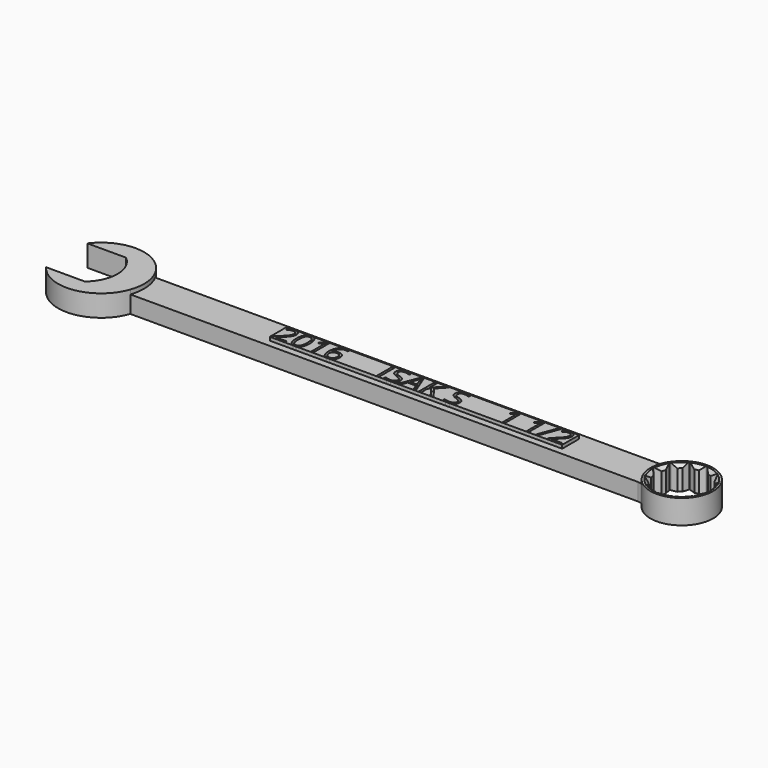
from build123d import *

# Parameters (mm, degrees)
F0_W         = 0.4390429688
F0_H         = 3.7777539063
F0_TEXT_SIZE = 5.2916666667
F1_DEPTH     = 12.7
F2_DEPTH     = 15.875
F0_R         = 19.05
F3_DEPTH     = 17.78
F4_SIZE      = 2.54
F5_R         = 23.1775
F6_DEPTH     = 17.78
F7_DEPTH     = 17.78
F8_COUNT     = 12
F11_DEPTH    = 2.54


# Not quite as in the source:
# - Text() gives the source's letters only with a copy of the font that has no kerning and outlines rounded to 1/6400 em; it was checked with that copy


with BuildPart() as f1:
    # F0 (on Top) → F1 (new body)
    with BuildSketch(Plane.XY):
        with BuildLine():
            ThreePointArc((28.0246586732, -7.9809556568), (31.6571563563, -20.4771515881), (29.9713945913, -33.3809556568))
            Line((29.9713945913, -33.3809556568), (404.6339280202, -33.3809556568))
            ThreePointArc((404.6339280202, -33.3809556568), (406.3354190659, -33.6131596303), (407.9124713773, -34.2927892879))
            Line((407.9124713773, -34.2927892879), (410.7505330951, -36.0037903424))
            ThreePointArc((410.7505330951, -36.0037903424), (406.5998341239, -20.5575243331), (413.8953174208, -6.3240651947))
            Line((413.8953174208, -6.3240651947), (410.0995642824, -7.6337042455))
            ThreePointArc((410.0995642824, -7.6337042455), (409.078462267, -7.8935411268), (408.0284512048, -7.9809556568))
            Line((408.0284512048, -7.9809556568), (28.0246586732, -7.9809556568))
        make_face()
        with BuildLine():
            ThreePointArc((254.0400713214, -25.8320806663), (253.1382651208, -28.1269866729), (250.8660139713, -29.0844430512))
            Line((250.8660139713, -29.0844430512), (144.2758794034, -29.0844430512))
            ThreePointArc((144.2758794034, -29.0844430512), (142.0308153732, -28.1545070815), (141.1008794034, -25.9094430512))
            Line((141.1008794034, -25.9094430512), (141.1008794034, -22.0994430512))
            ThreePointArc((141.1008794034, -22.0994430512), (142.0308153732, -19.854379021), (144.2758794034, -18.9244430512))
            Line((144.2758794034, -18.9244430512), (250.7731515389, -18.9244430512))
            ThreePointArc((250.7731515389, -18.9244430512), (252.9906951605, -19.8271919018), (253.9472088889, -22.0220806663))
            Line((253.9472088889, -22.0220806663), (254.0400713214, -25.8320806663))
        make_face(mode=Mode.SUBTRACT)
        with BuildLine():
            Line((144.2758794034, -29.0844430512), (250.8660139713, -29.0844430512))
            ThreePointArc((250.8660139713, -29.0844430512), (253.1382651208, -28.1269866729), (254.0400713214, -25.8320806663))
            Line((254.0400713214, -25.8320806663), (253.9472088889, -22.0220806663))
            ThreePointArc((253.9472088889, -22.0220806663), (252.9906951605, -19.8271919018), (250.7731515389, -18.9244430512))
            Line((250.7731515389, -18.9244430512), (144.2758794034, -18.9244430512))
            ThreePointArc((144.2758794034, -18.9244430512), (142.0308153732, -19.854379021), (141.1008794034, -22.0994430512))
            Line((141.1008794034, -22.0994430512), (141.1008794034, -25.9094430512))
            ThreePointArc((141.1008794034, -25.9094430512), (142.0308153732, -28.1545070815), (144.2758794034, -29.0844430512))
        make_face()
        with BuildLine():
            Line((147.0176241951, -25.5117412283), (147.0176241951, -25.9094430512))
            Line((147.0176241951, -25.9094430512), (144.5346749764, -25.9094430512))
            Line((144.5346749764, -25.9094430512), (144.5346749764, -25.5398532075))
            Line((144.5346749764, -25.5398532075), (145.5293429451, -24.5402243012))
            add(Edge.make_bspline(
                [(145.5293429451, -24.5402243012), (145.9840955493, -24.0796839366), (146.1287895597, -23.8833134939)],
                knots=[0, 0, 0, 1, 1, 1], degree=2))
            add(Edge.make_bspline(
                [(146.1287895597, -23.8833134939), (146.2734835701, -23.6869430512), (146.3458305753, -23.500907895)],
                knots=[0, 0, 0, 1, 1, 1], degree=2))
            add(Edge.make_bspline(
                [(146.3458305753, -23.500907895), (146.4181775805, -23.3148727387), (146.4181775805, -23.1007256033)],
                knots=[0, 0, 0, 1, 1, 1], degree=2))
            add(Edge.make_bspline(
                [(146.4181775805, -23.1007256033), (146.4181775805, -22.7981084158), (146.234622893, -22.6211683116)],
                knots=[0, 0, 0, 1, 1, 1], degree=2))
            add(Edge.make_bspline(
                [(146.234622893, -22.6211683116), (146.0510682055, -22.4442282075), (145.7252999764, -22.4442282075)],
                knots=[0, 0, 0, 1, 1, 1], degree=2))
            add(Edge.make_bspline(
                [(145.7252999764, -22.4442282075), (145.490482268, -22.4442282075), (145.2796424243, -22.5219495616)],
                knots=[0, 0, 0, 1, 1, 1], degree=2))
            add(Edge.make_bspline(
                [(145.2796424243, -22.5219495616), (145.0688025805, -22.5996709158), (144.8108338305, -22.8038961762)],
                knots=[0, 0, 0, 1, 1, 1], degree=2))
            Line((144.8108338305, -22.8038961762), (144.5834575284, -22.5120276866))
            add(Edge.make_bspline(
                [(144.5834575284, -22.5120276866), (145.1051827889, -22.0779456554), (145.7203390389, -22.0779456554)],
                knots=[0, 0, 0, 1, 1, 1], degree=2))
            add(Edge.make_bspline(
                [(145.7203390389, -22.0779456554), (146.2528129972, -22.0779456554), (146.5550167732, -22.3503838064)],
                knots=[0, 0, 0, 1, 1, 1], degree=2))
            add(Edge.make_bspline(
                [(146.5550167732, -22.3503838064), (146.8572205493, -22.6228219575), (146.8572205493, -23.0825354991)],
                knots=[0, 0, 0, 1, 1, 1], degree=2))
            add(Edge.make_bspline(
                [(146.8572205493, -23.0825354991), (146.8572205493, -23.4422034679), (146.6554757576, -23.7936032075)],
                knots=[0, 0, 0, 1, 1, 1], degree=2))
            add(Edge.make_bspline(
                [(146.6554757576, -23.7936032075), (146.4537309659, -24.1450029471), (145.9014132576, -24.6824378429)],
                knots=[0, 0, 0, 1, 1, 1], degree=2))
            Line((145.9014132576, -24.6824378429), (145.0745903409, -25.4910706554))
            Line((145.0745903409, -25.4910706554), (145.0745903409, -25.5117412283))
            Line((145.0745903409, -25.5117412283), (147.0176241951, -25.5117412283))
        make_face(mode=Mode.SUBTRACT)
        with BuildLine():
            add(Edge.make_bspline(
                [(149.7444861743, -22.5711455252), (150.0636398201, -23.0701331554), (150.0636398201, -24.0151917491)],
                knots=[0, 0, 0, 1, 1, 1], degree=2))
            add(Edge.make_bspline(
                [(150.0636398201, -24.0151917491), (150.0636398201, -24.9949769054), (149.7548214607, -25.4782549002)],
                knots=[0, 0, 0, 1, 1, 1], degree=2))
            add(Edge.make_bspline(
                [(149.7548214607, -25.4782549002), (149.4460031014, -25.961532895), (148.8101762784, -25.961532895)],
                knots=[0, 0, 0, 1, 1, 1], degree=2))
            add(Edge.make_bspline(
                [(148.8101762784, -25.961532895), (148.2008077889, -25.961532895), (147.8828943774, -25.4666793793)],
                knots=[0, 0, 0, 1, 1, 1], degree=2))
            add(Edge.make_bspline(
                [(147.8828943774, -25.4666793793), (147.5649809659, -24.9718258637), (147.5649809659, -24.0151917491)],
                knots=[0, 0, 0, 1, 1, 1], degree=2))
            add(Edge.make_bspline(
                [(147.5649809659, -24.0151917491), (147.5649809659, -23.0287920096), (147.8725590909, -22.5504749523)],
                knots=[0, 0, 0, 1, 1, 1], degree=2))
            add(Edge.make_bspline(
                [(147.8725590909, -22.5504749523), (148.1801372159, -22.072157895), (148.8101762784, -22.072157895)],
                knots=[0, 0, 0, 1, 1, 1], degree=2))
            add(Edge.make_bspline(
                [(148.8101762784, -22.072157895), (149.4253325284, -22.072157895), (149.7444861743, -22.5711455252)],
                knots=[0, 0, 0, 1, 1, 1], degree=2))
        make_face(mode=Mode.SUBTRACT)
        with BuildLine():
            Line((152.1736919034, -22.131689145), (152.1736919034, -25.9094430512))
            Line((152.1736919034, -25.9094430512), (151.7553195076, -25.9094430512))
            Line((151.7553195076, -25.9094430512), (151.7553195076, -23.2173076346))
            add(Edge.make_bspline(
                [(151.7553195076, -23.2173076346), (151.7553195076, -22.8807907075), (151.7759900805, -22.5814808116)],
                knots=[0, 0, 0, 1, 1, 1], degree=2))
            add(Edge.make_bspline(
                [(151.7759900805, -22.5814808116), (151.7222465909, -22.6360511241), (151.6548605232, -22.6951689627)],
                knots=[0, 0, 0, 1, 1, 1], degree=2))
            add(Edge.make_bspline(
                [(151.6548605232, -22.6951689627), (151.5874744555, -22.7542868012), (151.0401176847, -23.1991175304)],
                knots=[0, 0, 0, 1, 1, 1], degree=2))
            Line((151.0401176847, -23.1991175304), (150.8127413826, -22.9047685721))
            Line((150.8127413826, -22.9047685721), (151.8123702889, -22.131689145))
            Line((151.8123702889, -22.131689145), (152.1736919034, -22.131689145))
        make_face(mode=Mode.SUBTRACT)
        with BuildLine():
            add(Edge.make_bspline(
                [(153.9980766691, -25.5208362804), (153.6545317472, -25.0801396658), (153.6545317472, -24.294657895)],
                knots=[0, 0, 0, 1, 1, 1], degree=2))
            add(Edge.make_bspline(
                [(153.6545317472, -24.294657895), (153.6545317472, -23.1809274262), (154.0873735441, -22.6294365408)],
                knots=[0, 0, 0, 1, 1, 1], degree=2))
            add(Edge.make_bspline(
                [(154.0873735441, -22.6294365408), (154.5202153409, -22.0779456554), (155.3677088305, -22.0779456554)],
                knots=[0, 0, 0, 1, 1, 1], degree=2))
            add(Edge.make_bspline(
                [(155.3677088305, -22.0779456554), (155.6595773201, -22.0779456554), (155.8274223722, -22.1267282075)],
                knots=[0, 0, 0, 1, 1, 1], degree=2))
            Line((155.8274223722, -22.1267282075), (155.8274223722, -22.4963180512))
            add(Edge.make_bspline(
                [(155.8274223722, -22.4963180512), (155.6281580493, -22.4318258637), (155.372669768, -22.4318258637)],
                knots=[0, 0, 0, 1, 1, 1], degree=2))
            add(Edge.make_bspline(
                [(155.372669768, -22.4318258637), (154.7649549243, -22.4318258637), (154.4445610441, -22.8100973481)],
                knots=[0, 0, 0, 1, 1, 1], degree=2))
            add(Edge.make_bspline(
                [(154.4445610441, -22.8100973481), (154.1241671639, -23.1883688325), (154.0935747159, -24.0003089366)],
                knots=[0, 0, 0, 1, 1, 1], degree=2))
            Line((154.0935747159, -24.0003089366), (154.1241671639, -24.0003089366))
            add(Edge.make_bspline(
                [(154.1241671639, -24.0003089366), (154.4085942472, -23.5554782075), (155.0237504972, -23.5554782075)],
                knots=[0, 0, 0, 1, 1, 1], degree=2))
            add(Edge.make_bspline(
                [(155.0237504972, -23.5554782075), (155.5330734139, -23.5554782075), (155.8261821378, -23.8630563325)],
                knots=[0, 0, 0, 1, 1, 1], degree=2))
            add(Edge.make_bspline(
                [(155.8261821378, -23.8630563325), (156.1192908618, -24.1706344575), (156.1192908618, -24.6973206554)],
                knots=[0, 0, 0, 1, 1, 1], degree=2))
            add(Edge.make_bspline(
                [(156.1192908618, -24.6973206554), (156.1192908618, -25.286845395), (155.7976567472, -25.624189145)],
                knots=[0, 0, 0, 1, 1, 1], degree=2))
            add(Edge.make_bspline(
                [(155.7976567472, -25.624189145), (155.4760226326, -25.961532895), (154.9278390389, -25.961532895)],
                knots=[0, 0, 0, 1, 1, 1], degree=2))
            add(Edge.make_bspline(
                [(154.9278390389, -25.961532895), (154.3416215909, -25.961532895), (153.9980766691, -25.5208362804)],
                knots=[0, 0, 0, 1, 1, 1], degree=2))
        make_face(mode=Mode.SUBTRACT)
        with Locations((191.4911886482, -24.0205660981)):
            Rectangle(F0_W, F0_H, mode=Mode.SUBTRACT)
        with BuildLine():
            add(Edge.make_bspline(
                [(194.6550265389, -24.2739873221), (194.8782687264, -24.5170732596), (194.8782687264, -24.9040263846)],
                knots=[0, 0, 0, 1, 1, 1], degree=2))
            add(Edge.make_bspline(
                [(194.8782687264, -24.9040263846), (194.8782687264, -25.4026006033), (194.5165337003, -25.6820667491)],
                knots=[0, 0, 0, 1, 1, 1], degree=2))
            add(Edge.make_bspline(
                [(194.5165337003, -25.6820667491), (194.1547986743, -25.961532895), (193.5346814868, -25.961532895)],
                knots=[0, 0, 0, 1, 1, 1], degree=2))
            add(Edge.make_bspline(
                [(193.5346814868, -25.961532895), (192.8633012784, -25.961532895), (192.5011528409, -25.7879000825)],
                knots=[0, 0, 0, 1, 1, 1], degree=2))
            Line((192.5011528409, -25.7879000825), (192.5011528409, -25.3645667491))
            add(Edge.make_bspline(
                [(192.5011528409, -25.3645667491), (192.7343169034, -25.4621318533), (193.0079952889, -25.5191826346)],
                knots=[0, 0, 0, 1, 1, 1], degree=2))
            add(Edge.make_bspline(
                [(193.0079952889, -25.5191826346), (193.2816736743, -25.5762334158), (193.5503911222, -25.5762334158)],
                knots=[0, 0, 0, 1, 1, 1], degree=2))
            add(Edge.make_bspline(
                [(193.5503911222, -25.5762334158), (193.9894340909, -25.5762334158), (194.2118494555, -25.4096285981)],
                knots=[0, 0, 0, 1, 1, 1], degree=2))
            add(Edge.make_bspline(
                [(194.2118494555, -25.4096285981), (194.4342648201, -25.2430237804), (194.4342648201, -24.9453675304)],
                knots=[0, 0, 0, 1, 1, 1], degree=2))
            add(Edge.make_bspline(
                [(194.4342648201, -24.9453675304), (194.4342648201, -24.7494104991), (194.3553032316, -24.6241468273)],
                knots=[0, 0, 0, 1, 1, 1], degree=2))
            add(Edge.make_bspline(
                [(194.3553032316, -24.6241468273), (194.276341643, -24.4988831554), (194.0915467211, -24.3926364106)],
                knots=[0, 0, 0, 1, 1, 1], degree=2))
            add(Edge.make_bspline(
                [(194.0915467211, -24.3926364106), (193.9067517993, -24.2863896658), (193.5297205493, -24.1524443533)],
                knots=[0, 0, 0, 1, 1, 1], degree=2))
            add(Edge.make_bspline(
                [(193.5297205493, -24.1524443533), (193.0030343514, -23.9639287283), (192.7768982836, -23.7055465668)],
                knots=[0, 0, 0, 1, 1, 1], degree=2))
            add(Edge.make_bspline(
                [(192.7768982836, -23.7055465668), (192.5507622159, -23.4471644054), (192.5507622159, -23.0312724783)],
                knots=[0, 0, 0, 1, 1, 1], degree=2))
            add(Edge.make_bspline(
                [(192.5507622159, -23.0312724783), (192.5507622159, -22.5947099783), (192.8785975024, -22.3363278168)],
                knots=[0, 0, 0, 1, 1, 1], degree=2))
            add(Edge.make_bspline(
                [(192.8785975024, -22.3363278168), (193.2064327889, -22.0779456554), (193.7471749764, -22.0779456554)],
                knots=[0, 0, 0, 1, 1, 1], degree=2))
            add(Edge.make_bspline(
                [(193.7471749764, -22.0779456554), (194.3102413826, -22.0779456554), (194.7831840909, -22.2846513846)],
                knots=[0, 0, 0, 1, 1, 1], degree=2))
            Line((194.7831840909, -22.2846513846), (194.6459314868, -22.6666435721))
            add(Edge.make_bspline(
                [(194.6459314868, -22.6666435721), (194.1779497159, -22.4706865408), (193.7364262784, -22.4706865408)],
                knots=[0, 0, 0, 1, 1, 1], degree=2))
            add(Edge.make_bspline(
                [(193.7364262784, -22.4706865408), (193.3875070076, -22.4706865408), (193.1911365649, -22.6203414887)],
                knots=[0, 0, 0, 1, 1, 1], degree=2))
            add(Edge.make_bspline(
                [(193.1911365649, -22.6203414887), (192.9947661222, -22.7699964366), (192.9947661222, -23.0362334158)],
                knots=[0, 0, 0, 1, 1, 1], degree=2))
            add(Edge.make_bspline(
                [(192.9947661222, -23.0362334158), (192.9947661222, -23.2321904471), (193.0671131274, -23.3578675304)],
                knots=[0, 0, 0, 1, 1, 1], degree=2))
            add(Edge.make_bspline(
                [(193.0671131274, -23.3578675304), (193.1394601326, -23.4835446137), (193.3114392993, -23.5881377127)],
                knots=[0, 0, 0, 1, 1, 1], degree=2))
            add(Edge.make_bspline(
                [(193.3114392993, -23.5881377127), (193.4834184659, -23.6927308116), (193.8372986743, -23.8192347179)],
                knots=[0, 0, 0, 1, 1, 1], degree=2))
            add(Edge.make_bspline(
                [(193.8372986743, -23.8192347179), (194.4317843514, -24.0309013846), (194.6550265389, -24.2739873221)],
                knots=[0, 0, 0, 1, 1, 1], degree=2))
        make_face(mode=Mode.SUBTRACT)
        Polygon((198.4807361743, -25.9094430512), (198.0259835701, -25.9094430512), (197.5555213305, -24.7080693533), (196.0416085701, -24.7080693533), (195.5769340909, -25.9094430512), (195.1321033618, -25.9094430512), (196.6253455493, -22.1159795096), (196.994935393, -22.1159795096), align=None, mode=Mode.SUBTRACT)
        Polygon((200.1525721118, -23.7729326346), (201.7284965909, -25.9094430512), (201.211732268, -25.9094430512), (199.8350721118, -24.0772034679), (199.4390239347, -24.4286032075), (199.4390239347, -25.9094430512), (198.9999809659, -25.9094430512), (198.9999809659, -22.131689145), (199.4390239347, -22.131689145), (199.4390239347, -24.0052698741), (201.152201018, -22.131689145), (201.6714458097, -22.131689145), align=None, mode=Mode.SUBTRACT)
        with BuildLine():
            add(Edge.make_bspline(
                [(205.5310551847, -24.2739873221), (205.7542973722, -24.5170732596), (205.7542973722, -24.9040263846)],
                knots=[0, 0, 0, 1, 1, 1], degree=2))
            add(Edge.make_bspline(
                [(205.7542973722, -24.9040263846), (205.7542973722, -25.4026006033), (205.3925623461, -25.6820667491)],
                knots=[0, 0, 0, 1, 1, 1], degree=2))
            add(Edge.make_bspline(
                [(205.3925623461, -25.6820667491), (205.0308273201, -25.961532895), (204.4107101326, -25.961532895)],
                knots=[0, 0, 0, 1, 1, 1], degree=2))
            add(Edge.make_bspline(
                [(204.4107101326, -25.961532895), (203.7393299243, -25.961532895), (203.3771814868, -25.7879000825)],
                knots=[0, 0, 0, 1, 1, 1], degree=2))
            Line((203.3771814868, -25.7879000825), (203.3771814868, -25.3645667491))
            add(Edge.make_bspline(
                [(203.3771814868, -25.3645667491), (203.6103455493, -25.4621318533), (203.8840239347, -25.5191826346)],
                knots=[0, 0, 0, 1, 1, 1], degree=2))
            add(Edge.make_bspline(
                [(203.8840239347, -25.5191826346), (204.1577023201, -25.5762334158), (204.426419768, -25.5762334158)],
                knots=[0, 0, 0, 1, 1, 1], degree=2))
            add(Edge.make_bspline(
                [(204.426419768, -25.5762334158), (204.8654627368, -25.5762334158), (205.0878781014, -25.4096285981)],
                knots=[0, 0, 0, 1, 1, 1], degree=2))
            add(Edge.make_bspline(
                [(205.0878781014, -25.4096285981), (205.3102934659, -25.2430237804), (205.3102934659, -24.9453675304)],
                knots=[0, 0, 0, 1, 1, 1], degree=2))
            add(Edge.make_bspline(
                [(205.3102934659, -24.9453675304), (205.3102934659, -24.7494104991), (205.2313318774, -24.6241468273)],
                knots=[0, 0, 0, 1, 1, 1], degree=2))
            add(Edge.make_bspline(
                [(205.2313318774, -24.6241468273), (205.1523702889, -24.4988831554), (204.967575367, -24.3926364106)],
                knots=[0, 0, 0, 1, 1, 1], degree=2))
            add(Edge.make_bspline(
                [(204.967575367, -24.3926364106), (204.7827804451, -24.2863896658), (204.4057491951, -24.1524443533)],
                knots=[0, 0, 0, 1, 1, 1], degree=2))
            add(Edge.make_bspline(
                [(204.4057491951, -24.1524443533), (203.8790629972, -23.9639287283), (203.6529269295, -23.7055465668)],
                knots=[0, 0, 0, 1, 1, 1], degree=2))
            add(Edge.make_bspline(
                [(203.6529269295, -23.7055465668), (203.4267908618, -23.4471644054), (203.4267908618, -23.0312724783)],
                knots=[0, 0, 0, 1, 1, 1], degree=2))
            add(Edge.make_bspline(
                [(203.4267908618, -23.0312724783), (203.4267908618, -22.5947099783), (203.7546261482, -22.3363278168)],
                knots=[0, 0, 0, 1, 1, 1], degree=2))
            add(Edge.make_bspline(
                [(203.7546261482, -22.3363278168), (204.0824614347, -22.0779456554), (204.6232036222, -22.0779456554)],
                knots=[0, 0, 0, 1, 1, 1], degree=2))
            add(Edge.make_bspline(
                [(204.6232036222, -22.0779456554), (205.1862700284, -22.0779456554), (205.6592127368, -22.2846513846)],
                knots=[0, 0, 0, 1, 1, 1], degree=2))
            Line((205.6592127368, -22.2846513846), (205.5219601326, -22.6666435721))
            add(Edge.make_bspline(
                [(205.5219601326, -22.6666435721), (205.0539783618, -22.4706865408), (204.6124549243, -22.4706865408)],
                knots=[0, 0, 0, 1, 1, 1], degree=2))
            add(Edge.make_bspline(
                [(204.6124549243, -22.4706865408), (204.2635356534, -22.4706865408), (204.0671652107, -22.6203414887)],
                knots=[0, 0, 0, 1, 1, 1], degree=2))
            add(Edge.make_bspline(
                [(204.0671652107, -22.6203414887), (203.870794768, -22.7699964366), (203.870794768, -23.0362334158)],
                knots=[0, 0, 0, 1, 1, 1], degree=2))
            add(Edge.make_bspline(
                [(203.870794768, -23.0362334158), (203.870794768, -23.2321904471), (203.9431417732, -23.3578675304)],
                knots=[0, 0, 0, 1, 1, 1], degree=2))
            add(Edge.make_bspline(
                [(203.9431417732, -23.3578675304), (204.0154887784, -23.4835446137), (204.1874679451, -23.5881377127)],
                knots=[0, 0, 0, 1, 1, 1], degree=2))
            add(Edge.make_bspline(
                [(204.1874679451, -23.5881377127), (204.3594471118, -23.6927308116), (204.7133273201, -23.8192347179)],
                knots=[0, 0, 0, 1, 1, 1], degree=2))
            add(Edge.make_bspline(
                [(204.7133273201, -23.8192347179), (205.3078129972, -24.0309013846), (205.5310551847, -24.2739873221)],
                knots=[0, 0, 0, 1, 1, 1], degree=2))
        make_face(mode=Mode.SUBTRACT)
        with BuildLine():
            Line((238.1053976326, -22.131689145), (238.1053976326, -25.9094430512))
            Line((238.1053976326, -25.9094430512), (237.6870252368, -25.9094430512))
            Line((237.6870252368, -25.9094430512), (237.6870252368, -23.2173076346))
            add(Edge.make_bspline(
                [(237.6870252368, -23.2173076346), (237.6870252368, -22.8807907075), (237.7076958097, -22.5814808116)],
                knots=[0, 0, 0, 1, 1, 1], degree=2))
            add(Edge.make_bspline(
                [(237.7076958097, -22.5814808116), (237.6539523201, -22.6360511241), (237.5865662524, -22.6951689627)],
                knots=[0, 0, 0, 1, 1, 1], degree=2))
            add(Edge.make_bspline(
                [(237.5865662524, -22.6951689627), (237.5191801847, -22.7542868012), (236.9718234139, -23.1991175304)],
                knots=[0, 0, 0, 1, 1, 1], degree=2))
            Line((236.9718234139, -23.1991175304), (236.7444471118, -22.9047685721))
            Line((236.7444471118, -22.9047685721), (237.744076018, -22.131689145))
            Line((237.744076018, -22.131689145), (238.1053976326, -22.131689145))
        make_face(mode=Mode.SUBTRACT)
        with BuildLine():
            Line((242.5057491951, -22.131689145), (242.5057491951, -25.9094430512))
            Line((242.5057491951, -25.9094430512), (242.0873767993, -25.9094430512))
            Line((242.0873767993, -25.9094430512), (242.0873767993, -23.2173076346))
            add(Edge.make_bspline(
                [(242.0873767993, -23.2173076346), (242.0873767993, -22.8807907075), (242.1080473722, -22.5814808116)],
                knots=[0, 0, 0, 1, 1, 1], degree=2))
            add(Edge.make_bspline(
                [(242.1080473722, -22.5814808116), (242.0543038826, -22.6360511241), (241.9869178149, -22.6951689627)],
                knots=[0, 0, 0, 1, 1, 1], degree=2))
            add(Edge.make_bspline(
                [(241.9869178149, -22.6951689627), (241.9195317472, -22.7542868012), (241.3721749764, -23.1991175304)],
                knots=[0, 0, 0, 1, 1, 1], degree=2))
            Line((241.3721749764, -23.1991175304), (241.1447986743, -22.9047685721))
            Line((241.1447986743, -22.9047685721), (242.1444275805, -22.131689145))
            Line((242.1444275805, -22.131689145), (242.5057491951, -22.131689145))
        make_face(mode=Mode.SUBTRACT)
        Polygon((245.1441411222, -22.131689145), (245.572435393, -22.131689145), (244.1643559659, -25.9094430512), (243.7360616951, -25.9094430512), align=None, mode=Mode.SUBTRACT)
        with BuildLine():
            Line((248.3687504972, -25.5117412283), (248.3687504972, -25.9094430512))
            Line((248.3687504972, -25.9094430512), (245.8858012784, -25.9094430512))
            Line((245.8858012784, -25.9094430512), (245.8858012784, -25.5398532075))
            Line((245.8858012784, -25.5398532075), (246.8804692472, -24.5402243012))
            add(Edge.make_bspline(
                [(246.8804692472, -24.5402243012), (247.3352218514, -24.0796839366), (247.4799158618, -23.8833134939)],
                knots=[0, 0, 0, 1, 1, 1], degree=2))
            add(Edge.make_bspline(
                [(247.4799158618, -23.8833134939), (247.6246098722, -23.6869430512), (247.6969568774, -23.500907895)],
                knots=[0, 0, 0, 1, 1, 1], degree=2))
            add(Edge.make_bspline(
                [(247.6969568774, -23.500907895), (247.7693038826, -23.3148727387), (247.7693038826, -23.1007256033)],
                knots=[0, 0, 0, 1, 1, 1], degree=2))
            add(Edge.make_bspline(
                [(247.7693038826, -23.1007256033), (247.7693038826, -22.7981084158), (247.5857491951, -22.6211683116)],
                knots=[0, 0, 0, 1, 1, 1], degree=2))
            add(Edge.make_bspline(
                [(247.5857491951, -22.6211683116), (247.4021945076, -22.4442282075), (247.0764262784, -22.4442282075)],
                knots=[0, 0, 0, 1, 1, 1], degree=2))
            add(Edge.make_bspline(
                [(247.0764262784, -22.4442282075), (246.8416085701, -22.4442282075), (246.6307687264, -22.5219495616)],
                knots=[0, 0, 0, 1, 1, 1], degree=2))
            add(Edge.make_bspline(
                [(246.6307687264, -22.5219495616), (246.4199288826, -22.5996709158), (246.1619601326, -22.8038961762)],
                knots=[0, 0, 0, 1, 1, 1], degree=2))
            Line((246.1619601326, -22.8038961762), (245.9345838305, -22.5120276866))
            add(Edge.make_bspline(
                [(245.9345838305, -22.5120276866), (246.4563090909, -22.0779456554), (247.0714653409, -22.0779456554)],
                knots=[0, 0, 0, 1, 1, 1], degree=2))
            add(Edge.make_bspline(
                [(247.0714653409, -22.0779456554), (247.6039392993, -22.0779456554), (247.9061430753, -22.3503838064)],
                knots=[0, 0, 0, 1, 1, 1], degree=2))
            add(Edge.make_bspline(
                [(247.9061430753, -22.3503838064), (248.2083468514, -22.6228219575), (248.2083468514, -23.0825354991)],
                knots=[0, 0, 0, 1, 1, 1], degree=2))
            add(Edge.make_bspline(
                [(248.2083468514, -23.0825354991), (248.2083468514, -23.4422034679), (248.0066020597, -23.7936032075)],
                knots=[0, 0, 0, 1, 1, 1], degree=2))
            add(Edge.make_bspline(
                [(248.0066020597, -23.7936032075), (247.804857268, -24.1450029471), (247.2525395597, -24.6824378429)],
                knots=[0, 0, 0, 1, 1, 1], degree=2))
            Line((247.2525395597, -24.6824378429), (246.425716643, -25.4910706554))
            Line((246.425716643, -25.4910706554), (246.425716643, -25.5117412283))
            Line((246.425716643, -25.5117412283), (248.3687504972, -25.5117412283))
        make_face(mode=Mode.SUBTRACT)
        Polygon((248.9963090909, -22.131689145), (249.4766932055, -22.131689145), (249.3733403409, -23.4959469575), (249.1021424243, -23.4959469575), align=None, mode=Mode.SUBTRACT)
        Polygon((249.9496359139, -22.131689145), (250.4300200284, -22.131689145), (250.3241866951, -23.4959469575), (250.0554692472, -23.4959469575), align=None, mode=Mode.SUBTRACT)
        with BuildLine():
            add(Edge.make_bspline(
                [(148.1929529711, -22.8175387543), (147.9990629972, -23.1908493012), (147.9990629972, -24.0151917491)],
                knots=[0, 0, 0, 1, 1, 1], degree=2))
            add(Edge.make_bspline(
                [(147.9990629972, -24.0151917491), (147.9990629972, -24.8395341971), (148.1929529711, -25.2157386241)],
                knots=[0, 0, 0, 1, 1, 1], degree=2))
            add(Edge.make_bspline(
                [(148.1929529711, -25.2157386241), (148.3868429451, -25.5919430512), (148.8101762784, -25.5919430512)],
                knots=[0, 0, 0, 1, 1, 1], degree=2))
            add(Edge.make_bspline(
                [(148.8101762784, -25.5919430512), (149.2392973722, -25.5919430512), (149.4315337003, -25.2107776866)],
                knots=[0, 0, 0, 1, 1, 1], degree=2))
            add(Edge.make_bspline(
                [(149.4315337003, -25.2107776866), (149.6237700284, -24.8296123221), (149.6237700284, -24.0151917491)],
                knots=[0, 0, 0, 1, 1, 1], degree=2))
            add(Edge.make_bspline(
                [(149.6237700284, -24.0151917491), (149.6237700284, -23.2015979991), (149.4315337003, -22.8229131033)],
                knots=[0, 0, 0, 1, 1, 1], degree=2))
            add(Edge.make_bspline(
                [(149.4315337003, -22.8229131033), (149.2392973722, -22.4442282075), (148.8101762784, -22.4442282075)],
                knots=[0, 0, 0, 1, 1, 1], degree=2))
            add(Edge.make_bspline(
                [(148.8101762784, -22.4442282075), (148.3868429451, -22.4442282075), (148.1929529711, -22.8175387543)],
                knots=[0, 0, 0, 1, 1, 1], degree=2))
        make_face()
        with BuildLine():
            add(Edge.make_bspline(
                [(154.4900363045, -25.4625452648), (154.6797921639, -25.5969039887), (154.9228781014, -25.5969039887)],
                knots=[0, 0, 0, 1, 1, 1], degree=2))
            add(Edge.make_bspline(
                [(154.9228781014, -25.5969039887), (155.2899874764, -25.5969039887), (155.4925590909, -25.3653935721)],
                knots=[0, 0, 0, 1, 1, 1], degree=2))
            add(Edge.make_bspline(
                [(155.4925590909, -25.3653935721), (155.6951307055, -25.1338831554), (155.6951307055, -24.6973206554)],
                knots=[0, 0, 0, 1, 1, 1], degree=2))
            add(Edge.make_bspline(
                [(155.6951307055, -24.6973206554), (155.6951307055, -24.3227698741), (155.5066150805, -24.1082093273)],
                knots=[0, 0, 0, 1, 1, 1], degree=2))
            add(Edge.make_bspline(
                [(155.5066150805, -24.1082093273), (155.3180994555, -23.8936487804), (154.9435486743, -23.8936487804)],
                knots=[0, 0, 0, 1, 1, 1], degree=2))
            add(Edge.make_bspline(
                [(154.9435486743, -23.8936487804), (154.7112114347, -23.8936487804), (154.5173214607, -23.9895602387)],
                knots=[0, 0, 0, 1, 1, 1], degree=2))
            add(Edge.make_bspline(
                [(154.5173214607, -23.9895602387), (154.3234314868, -24.0854716971), (154.2085031014, -24.2533167491)],
                knots=[0, 0, 0, 1, 1, 1], degree=2))
            add(Edge.make_bspline(
                [(154.2085031014, -24.2533167491), (154.0935747159, -24.4211618012), (154.0935747159, -24.60223602)],
                knots=[0, 0, 0, 1, 1, 1], degree=2))
            add(Edge.make_bspline(
                [(154.0935747159, -24.60223602), (154.0935747159, -24.8684729991), (154.1969275805, -25.09832977)],
                knots=[0, 0, 0, 1, 1, 1], degree=2))
            add(Edge.make_bspline(
                [(154.1969275805, -25.09832977), (154.3002804451, -25.3281865408), (154.4900363045, -25.4625452648)],
                knots=[0, 0, 0, 1, 1, 1], degree=2))
        make_face()
        with BuildLine():
            Line((196.1970512784, -24.3128479991), (197.4190955493, -24.3128479991))
            Line((197.4190955493, -24.3128479991), (196.9792257576, -23.1420667491))
            add(Edge.make_bspline(
                [(196.9792257576, -23.1420667491), (196.8940629972, -22.9196513846), (196.8039392993, -22.5971904471)],
                knots=[0, 0, 0, 1, 1, 1], degree=2))
            add(Edge.make_bspline(
                [(196.8039392993, -22.5971904471), (196.746888518, -22.8452373221), (196.6410551847, -23.1420667491)],
                knots=[0, 0, 0, 1, 1, 1], degree=2))
            Line((196.6410551847, -23.1420667491), (196.1970512784, -24.3128479991))
        make_face()
        with Locations((144.2758794034, -25.9094430512)):
            Text('2016                         ISAK S                      1 1/2"', F0_TEXT_SIZE, font='Open Sans', text_align=(TextAlign.LEFT, TextAlign.BOTTOM))
    extrude(amount=F1_DEPTH)

    # F0 (on Top) → F2 (join)
    with BuildSketch(Plane.XY):
        with BuildLine():
            Line((3.175, -41.9534556568), (-25.4, -41.9534556568))
            ThreePointArc((-25.4, -41.9534556568), (4.8576075582, -54.2796592004), (29.9713945913, -33.3809556568))
            ThreePointArc((29.9713945913, -33.3809556568), (31.6571563563, -20.4771515881), (28.0246586732, -7.9809556568))
            ThreePointArc((28.0246586732, -7.9809556568), (2.4456639896, 8.7522109394), (-25.4, -3.8534556568))
            Line((-25.4, -3.8534556568), (3.175, -3.8534556568))
            ThreePointArc((3.175, -3.8534556568), (12.0699524055, -22.9034556568), (3.175, -41.9534556568))
        make_face()
    extrude(amount=F2_DEPTH)

    # F0 (on Top) → F3 (join)
    with BuildSketch(Plane.XY):
        with BuildLine():
            ThreePointArc((413.8953174208, -6.3240651947), (406.5998341239, -20.5575243331), (410.7505330951, -36.0037903424))
            ThreePointArc((410.7505330951, -36.0037903424), (435.5931010732, -44.0287078572), (450.9261153558, -22.899317003))
            ThreePointArc((450.9261153558, -22.899317003), (437.7810868837, -2.6137373452), (413.8953174208, -6.3240651947))
        make_face()
        with Locations((428.7011153558, -22.899317003)):
            Circle(F0_R, mode=Mode.SUBTRACT)
    extrude(amount=F3_DEPTH)

    # F4
    f4_edges = [f1.edges().sort_by_distance(p)[0] for p in [
        (409.651115, -22.899317, 17.78),
    ]]
    chamfer(f4_edges, length=F4_SIZE)

    # F5 (on face) → F6 (join)
    with BuildSketch(Plane.XY.offset(17.78)):
        with Locations((428.7011153558, -22.899317003)):
            Circle(F5_R)
        with BuildLine():
            ThreePointArc((406.6808373244, -19.8896691131), (407.6216405464, -15.8561382632), (409.2945158604, -12.0672109739))
            ThreePointArc((409.2945158604, -12.0672109739), (411.6413657407, -8.6544734423), (414.5806861024, -5.7364471177))
            ThreePointArc((414.5806861024, -5.7364471177), (418.0103968689, -3.4144725532), (421.811387125, -1.7691899351))
            ThreePointArc((421.811387125, -1.7691899351), (425.8101116486, -0.8631484938), (429.9072262122, -0.7070678695))
            ThreePointArc((429.9072262122, -0.7070678695), (433.9632929919, -1.3062599817), (437.8402711503, -2.6403324193))
            ThreePointArc((437.8402711503, -2.6403324193), (441.3718211102, -4.6399675982), (444.4808765864, -7.2484460846))
            ThreePointArc((444.4808765864, -7.2484460846), (447.1017278191, -10.4346434824), (449.0885246231, -14.0503527492))
            ThreePointArc((449.0885246231, -14.0503527492), (450.3644154805, -17.9342336498), (450.9073457293, -21.9861042147))
            ThreePointArc((450.9073457293, -21.9861042147), (450.9214224537, -22.4426141741), (450.9261153558, -22.899317003))
            ThreePointArc((450.9261153558, -22.899317003), (450.6176350497, -26.5894104307), (449.70075747, -30.1770677594))
            ThreePointArc((449.70075747, -30.1770677594), (448.0145461281, -33.8966810872), (445.6761937607, -37.2449552999))
            ThreePointArc((445.6761937607, -37.2449552999), (442.7646624402, -40.1088279897), (439.3782601188, -42.3916027774))
            ThreePointArc((439.3782601188, -42.3916027774), (435.6396794195, -44.0134580874), (431.6678132357, -44.9254226209))
            ThreePointArc((431.6678132357, -44.9254226209), (427.5784432253, -45.0959436), (423.5271479334, -44.5136799617))
            ThreePointArc((423.5271479334, -44.5136799617), (419.5902103807, -43.1710222972), (415.9724115332, -41.1182830548))
            ThreePointArc((415.9724115332, -41.1182830548), (412.8170374696, -38.4443063792), (410.2117620358, -35.2319744137))
            ThreePointArc((410.2117620358, -35.2319744137), (408.261002646, -31.6258522496), (407.0058384781, -27.7227583266))
            ThreePointArc((407.0058384781, -27.7227583266), (406.4952207125, -23.8206573812), (406.6808373244, -19.8896691131))
        make_face(mode=Mode.SUBTRACT)
    extrude(amount=-F6_DEPTH)


with BuildPart() as f7:
    # F5 (on face) → F7 (new body, through all)
    with BuildSketch(Plane.XY.offset(17.78)):
        with BuildLine():
            Line((429.2230926978, -1.315627799), (426.1875151916, -4.0158767917))
            ThreePointArc((426.1875151916, -4.0158767917), (429.6990692744, -3.8754743844), (433.1766598152, -4.3825137748))
            Line((433.1766598152, -4.3825137748), (430.5105105856, -1.3852706866))
            ThreePointArc((430.5105105856, -1.3852706866), (429.8673216198, -1.3408369325), (429.2230926978, -1.315627799))
        make_face()
        with BuildLine():
            Line((429.9072262122, -0.7070678695), (429.2230926978, -1.315627799))
            ThreePointArc((429.2230926978, -1.315627799), (429.8673216198, -1.3408369325), (430.5105105856, -1.3852706866))
            Line((430.5105105856, -1.3852706866), (429.9072262122, -0.7070678695))
        make_face()
    extrude(amount=-F7_DEPTH)


with BuildPart() as f8_1:
    # F8: instance of F7
    add(f7.part.rotate(Axis((428.7011153558, -22.899317003, 0), (0, 0, -1)), 1 * 360 / F8_COUNT))


with BuildPart() as f8_2:
    # F8: instance of F7
    add(f7.part.rotate(Axis((428.7011153558, -22.899317003, 0), (0, 0, -1)), 2 * 360 / F8_COUNT))


with BuildPart() as f8_3:
    # F8: instance of F7
    add(f7.part.rotate(Axis((428.7011153558, -22.899317003, 0), (0, 0, -1)), 3 * 360 / F8_COUNT))


with BuildPart() as f8_4:
    # F8: instance of F7
    add(f7.part.rotate(Axis((428.7011153558, -22.899317003, 0), (0, 0, -1)), 4 * 360 / F8_COUNT))


with BuildPart() as f8_5:
    # F8: instance of F7
    add(f7.part.rotate(Axis((428.7011153558, -22.899317003, 0), (0, 0, -1)), 5 * 360 / F8_COUNT))


with BuildPart() as f8_6:
    # F8: instance of F7
    add(f7.part.rotate(Axis((428.7011153558, -22.899317003, 0), (0, 0, -1)), 6 * 360 / F8_COUNT))


with BuildPart() as f8_7:
    # F8: instance of F7
    add(f7.part.rotate(Axis((428.7011153558, -22.899317003, 0), (0, 0, -1)), 7 * 360 / F8_COUNT))


with BuildPart() as f8_8:
    # F8: instance of F7
    add(f7.part.rotate(Axis((428.7011153558, -22.899317003, 0), (0, 0, -1)), 8 * 360 / F8_COUNT))


with BuildPart() as f8_9:
    # F8: instance of F7
    add(f7.part.rotate(Axis((428.7011153558, -22.899317003, 0), (0, 0, -1)), 9 * 360 / F8_COUNT))


with BuildPart() as f8_10:
    # F8: instance of F7
    add(f7.part.rotate(Axis((428.7011153558, -22.899317003, 0), (0, 0, -1)), 10 * 360 / F8_COUNT))


with BuildPart() as f8_11:
    # F8: instance of F7
    add(f7.part.rotate(Axis((428.7011153558, -22.899317003, 0), (0, 0, -1)), 11 * 360 / F8_COUNT))


with BuildPart() as f1_1:
    add(f1.part)

    # F9: cut F7, F8_1, F8_2, F8_3, F8_4, F8_5, F8_6, F8_7, F8_8, F8_9, F8_10, F8_11
    add(f7.part, mode=Mode.SUBTRACT)
    add(f8_1.part, mode=Mode.SUBTRACT)
    add(f8_2.part, mode=Mode.SUBTRACT)
    add(f8_3.part, mode=Mode.SUBTRACT)
    add(f8_4.part, mode=Mode.SUBTRACT)
    add(f8_5.part, mode=Mode.SUBTRACT)
    add(f8_6.part, mode=Mode.SUBTRACT)
    add(f8_7.part, mode=Mode.SUBTRACT)
    add(f8_8.part, mode=Mode.SUBTRACT)
    add(f8_9.part, mode=Mode.SUBTRACT)
    add(f8_10.part, mode=Mode.SUBTRACT)
    add(f8_11.part, mode=Mode.SUBTRACT)

    # F10 (on face) → F11 (join)
    with BuildSketch(Plane.XY.offset(12.7)):
        with BuildLine():
            Line((344.7478053731, -28.1739556568), (344.7478053731, -12.8160896817))
            Line((344.7478053731, -12.8160896817), (339.2679984715, -12.8160896817))
            add(Edge.make_bspline(
                [(339.2679984715, -12.8160896817), (340.6239472568, -13.0379191573), (341.4999233434, -13.8276157935)],
                knots=[0.2809046733, 0.2809046733, 0.2809046733, 1, 1, 1], degree=2))
            add(Edge.make_bspline(
                [(341.4999233434, -13.8276157935), (342.7180874089, -14.9257965311), (342.7180874089, -16.7788723736)],
                knots=[0, 0, 0, 1, 1, 1], degree=2))
            add(Edge.make_bspline(
                [(342.7180874089, -16.7788723736), (342.7180874089, -18.2286709194), (341.9048670751, -19.6451407631)],
                knots=[0, 0, 0, 1, 1, 1], degree=2))
            add(Edge.make_bspline(
                [(341.9048670751, -19.6451407631), (341.0916467414, -21.0616106067), (338.8652894342, -23.2279762499)],
                knots=[0, 0, 0, 1, 1, 1], degree=2))
            Line((338.8652894342, -23.2279762499), (335.532419214, -26.4875233253))
            Line((335.532419214, -26.4875233253), (335.532419214, -26.5708450808))
            Line((335.532419214, -26.5708450808), (343.3646642316, -26.5708450808))
            Line((343.3646642316, -26.5708450808), (343.3646642316, -28.1739556568))
            Line((343.3646642316, -28.1739556568), (344.7478053731, -28.1739556568))
        make_face()
        with BuildLine():
            Line((344.7478053731, -12.6890896817), (128.8478053731, -12.6890896817))
            Line((128.8478053731, -12.6890896817), (128.8478053731, -12.8160896817))
            Line((128.8478053731, -12.8160896817), (133.5853386769, -12.8160896817))
            add(Edge.make_bspline(
                [(133.5853386769, -12.8160896817), (134.1185084741, -12.729435056), (134.6703296479, -12.729435056)],
                knots=[0.7774605439, 0.7774605439, 0.7774605439, 1, 1, 1], degree=2))
            add(Edge.make_bspline(
                [(134.6703296479, -12.729435056), (135.2732545683, -12.729435056), (135.8029372634, -12.8160896817)],
                knots=[0, 0, 0, 0.2809046733, 0.2809046733, 0.2809046733], degree=2))
            Line((135.8029372634, -12.8160896817), (145.986278987, -12.8160896817))
            add(Edge.make_bspline(
                [(145.986278987, -12.8160896817), (146.5186988239, -12.7061049644), (147.1252656611, -12.7061049644)],
                knots=[0.7611609757, 0.7611609757, 0.7611609757, 1, 1, 1], degree=2))
            add(Edge.make_bspline(
                [(147.1252656611, -12.7061049644), (147.7051076631, -12.7061049644), (148.2197060383, -12.8160896817)],
                knots=[0, 0, 0, 0.2338397471, 0.2338397471, 0.2338397471], degree=2))
            Line((148.2197060383, -12.8160896817), (172.2744622205, -12.8160896817))
            add(Edge.make_bspline(
                [(172.2744622205, -12.8160896817), (172.8837841166, -12.729435056), (173.5582593782, -12.729435056)],
                knots=[0.802565176, 0.802565176, 0.802565176, 1, 1, 1], degree=2))
            add(Edge.make_bspline(
                [(173.5582593782, -12.729435056), (174.3392643102, -12.729435056), (174.8999608716, -12.8160896817)],
                knots=[0, 0, 0, 0.6638357975, 0.6638357975, 0.6638357975], degree=2))
            Line((174.8999608716, -12.8160896817), (216.226127589, -12.8160896817))
            add(Edge.make_bspline(
                [(216.226127589, -12.8160896817), (216.7834449571, -12.729435056), (217.4121657368, -12.729435056)],
                knots=[0.711555898, 0.711555898, 0.711555898, 1, 1, 1], degree=2))
            add(Edge.make_bspline(
                [(217.4121657368, -12.729435056), (218.1441170333, -12.729435056), (218.838286913, -12.8160896817)],
                knots=[0, 0, 0, 0.3224903099, 0.3224903099, 0.3224903099], degree=2))
            Line((218.838286913, -12.8160896817), (260.0667024667, -12.8160896817))
            add(Edge.make_bspline(
                [(260.0667024667, -12.8160896817), (260.6240198347, -12.729435056), (261.2527406144, -12.729435056)],
                knots=[0.711555898, 0.711555898, 0.711555898, 1, 1, 1], degree=2))
            add(Edge.make_bspline(
                [(261.2527406144, -12.729435056), (261.984691911, -12.729435056), (262.6788617907, -12.8160896817)],
                knots=[0, 0, 0, 0.3224903099, 0.3224903099, 0.3224903099], degree=2))
            Line((262.6788617907, -12.8160896817), (337.050399885, -12.8160896817))
            add(Edge.make_bspline(
                [(337.050399885, -12.8160896817), (337.5835696822, -12.729435056), (338.135390856, -12.729435056)],
                knots=[0.7774605439, 0.7774605439, 0.7774605439, 1, 1, 1], degree=2))
            add(Edge.make_bspline(
                [(338.135390856, -12.729435056), (338.7383157764, -12.729435056), (339.2679984715, -12.8160896817)],
                knots=[0, 0, 0, 0.2809046733, 0.2809046733, 0.2809046733], degree=2))
            Line((339.2679984715, -12.8160896817), (344.7478053731, -12.8160896817))
            Line((344.7478053731, -12.8160896817), (344.7478053731, -12.6890896817))
        make_face()
        with BuildLine():
            Line((133.5853386769, -12.8160896817), (128.8478053731, -12.8160896817))
            Line((128.8478053731, -12.8160896817), (128.8478053731, -28.1739556568))
            Line((128.8478053731, -28.1739556568), (129.890993752, -28.1739556568))
            Line((129.890993752, -28.1739556568), (129.890993752, -26.6841626683))
            Line((129.890993752, -26.6841626683), (133.900436627, -22.654722572))
            add(Edge.make_bspline(
                [(133.900436627, -22.654722572), (135.7335152482, -20.7983138593), (136.3167675367, -20.006757182)],
                knots=[0, 0, 0, 1, 1, 1], degree=2))
            add(Edge.make_bspline(
                [(136.3167675367, -20.006757182), (136.9000198253, -19.2152005046), (137.1916459695, -18.4653047051)],
                knots=[0, 0, 0, 1, 1, 1], degree=2))
            add(Edge.make_bspline(
                [(137.1916459695, -18.4653047051), (137.4832721138, -17.7154089055), (137.4832721138, -16.8521955185)],
                knots=[0, 0, 0, 1, 1, 1], degree=2))
            add(Edge.make_bspline(
                [(137.4832721138, -16.8521955185), (137.4832721138, -15.6323650178), (136.7433749249, -14.9191307907)],
                knots=[0, 0, 0, 1, 1, 1], degree=2))
            add(Edge.make_bspline(
                [(136.7433749249, -14.9191307907), (136.003477736, -14.2058965635), (134.6903268692, -14.2058965635)],
                knots=[0, 0, 0, 1, 1, 1], degree=2))
            add(Edge.make_bspline(
                [(134.6903268692, -14.2058965635), (133.7437917267, -14.2058965635), (132.8939098205, -14.5191863642)],
                knots=[0, 0, 0, 1, 1, 1], degree=2))
            add(Edge.make_bspline(
                [(132.8939098205, -14.5191863642), (132.0440279143, -14.832476165), (131.0041724056, -15.6556951094)],
                knots=[0, 0, 0, 1, 1, 1], degree=2))
            Line((131.0041724056, -15.6556951094), (130.087633095, -14.4791919216))
            add(Edge.make_bspline(
                [(130.087633095, -14.4791919216), (131.7226645794, -13.1188249972), (133.5853386769, -12.8160896817)],
                knots=[0, 0, 0, 0.7774605439, 0.7774605439, 0.7774605439], degree=2))
        make_face()
        with BuildLine():
            Line((129.890993752, -28.1739556568), (128.8478053731, -28.1739556568))
            Line((128.8478053731, -28.1739556568), (128.8478053731, -28.3009556568))
            Line((128.8478053731, -28.3009556568), (146.1722033543, -28.3009556568))
            add(Edge.make_bspline(
                [(146.1722033543, -28.3009556568), (145.9051022417, -28.2519361316), (145.65505833, -28.1739556568)],
                knots=[0.2039489259, 0.2039489259, 0.2039489259, 0.3244428423, 0.3244428423, 0.3244428423], degree=2))
            Line((145.65505833, -28.1739556568), (139.8996030235, -28.1739556568))
            Line((139.8996030235, -28.1739556568), (129.890993752, -28.1739556568))
        make_face()
        with BuildLine():
            Line((344.7478053731, -28.3009556568), (344.7478053731, -28.1739556568))
            Line((344.7478053731, -28.1739556568), (343.3646642316, -28.1739556568))
            Line((343.3646642316, -28.1739556568), (333.3560549601, -28.1739556568))
            Line((333.3560549601, -28.1739556568), (326.4170191615, -28.1739556568))
            Line((326.4170191615, -28.1739556568), (324.6905923874, -28.1739556568))
            Line((324.6905923874, -28.1739556568), (319.7312814996, -28.1739556568))
            Line((319.7312814996, -28.1739556568), (318.0448491681, -28.1739556568))
            Line((318.0448491681, -28.1739556568), (301.9937461872, -28.1739556568))
            Line((301.9937461872, -28.1739556568), (300.3073138557, -28.1739556568))
            Line((300.3073138557, -28.1739556568), (262.3604117209, -28.1739556568))
            add(Edge.make_bspline(
                [(262.3604117209, -28.1739556568), (262.031717543, -28.2519361316), (261.6762473391, -28.3009556568)],
                knots=[0.5682703015, 0.5682703015, 0.5682703015, 0.7286091822, 0.7286091822, 0.7286091822], degree=2))
            Line((261.6762473391, -28.3009556568), (344.7478053731, -28.3009556568))
        make_face()
        with BuildLine():
            add(Edge.make_bspline(
                [(146.1722033543, -28.3009556568), (145.9051022417, -28.2519361316), (145.65505833, -28.1739556568)],
                knots=[0.2039489259, 0.2039489259, 0.2039489259, 0.3244428423, 0.3244428423, 0.3244428423], degree=2))
            Line((146.1722033543, -28.3009556568), (148.1270026884, -28.3009556568))
            add(Edge.make_bspline(
                [(148.6660680686, -28.1739556568), (148.4063335441, -28.2519361316), (148.1270026884, -28.3009556568)],
                knots=[0.6716946069, 0.6716946069, 0.6716946069, 0.7936230252, 0.7936230252, 0.7936230252], degree=2))
            Line((148.6660680686, -28.1739556568), (145.65505833, -28.1739556568))
        make_face()
        with BuildLine():
            Line((148.1270026884, -28.3009556568), (146.1722033543, -28.3009556568))
            add(Edge.make_bspline(
                [(147.1252656611, -28.3839264806), (146.6243007438, -28.3839264806), (146.1722033543, -28.3009556568)],
                knots=[0, 0, 0, 0.2039489259, 0.2039489259, 0.2039489259], degree=2))
            add(Edge.make_bspline(
                [(148.1270026884, -28.3009556568), (147.6542051421, -28.3839264806), (147.1252656611, -28.3839264806)],
                knots=[0.7936230252, 0.7936230252, 0.7936230252, 1, 1, 1], degree=2))
        make_face()
        with BuildLine():
            add(Edge.make_bspline(
                [(261.6762473391, -28.3009556568), (261.0745757488, -28.3839264806), (260.3961929678, -28.3839264806)],
                knots=[0.7286091822, 0.7286091822, 0.7286091822, 1, 1, 1], degree=2))
            Line((261.6762473391, -28.3009556568), (258.6803790273, -28.3009556568))
            add(Edge.make_bspline(
                [(260.3961929678, -28.3839264806), (259.4644024544, -28.3839264806), (258.6803790273, -28.3009556568)],
                knots=[0, 0, 0, 0.3443054145, 0.3443054145, 0.3443054145], degree=2))
        make_face()
        with BuildLine():
            Line((258.6803790273, -28.3009556568), (261.6762473391, -28.3009556568))
            add(Edge.make_bspline(
                [(262.3604117209, -28.1739556568), (262.031717543, -28.2519361316), (261.6762473391, -28.3009556568)],
                knots=[0.5682703015, 0.5682703015, 0.5682703015, 0.7286091822, 0.7286091822, 0.7286091822], degree=2))
            Line((262.3604117209, -28.1739556568), (257.8055481683, -28.1739556568))
            add(Edge.make_bspline(
                [(258.6803790273, -28.3009556568), (258.2171745617, -28.2519361316), (257.8055481683, -28.1739556568)],
                knots=[0.3443054145, 0.3443054145, 0.3443054145, 0.5477225575, 0.5477225575, 0.5477225575], degree=2))
        make_face()
        with BuildLine():
            add(Edge.make_bspline(
                [(148.6660680686, -28.1739556568), (148.4063335441, -28.2519361316), (148.1270026884, -28.3009556568)],
                knots=[0.6716946069, 0.6716946069, 0.6716946069, 0.7936230252, 0.7936230252, 0.7936230252], degree=2))
            Line((148.1270026884, -28.3009556568), (170.8094874911, -28.3009556568))
            add(Edge.make_bspline(
                [(170.8094874911, -28.3009556568), (170.5347644957, -28.2519361316), (170.2759890402, -28.1739556568)],
                knots=[0.2161174802, 0.2161174802, 0.2161174802, 0.3438006316, 0.3438006316, 0.3438006316], degree=2))
            Line((170.2759890402, -28.1739556568), (160.6833817172, -28.1739556568))
            Line((160.6833817172, -28.1739556568), (158.9969493858, -28.1739556568))
            Line((158.9969493858, -28.1739556568), (148.6660680686, -28.1739556568))
        make_face()
        with BuildLine():
            Line((217.8356724615, -28.3009556568), (258.6803790273, -28.3009556568))
            add(Edge.make_bspline(
                [(258.6803790273, -28.3009556568), (258.2171745617, -28.2519361316), (257.8055481683, -28.1739556568)],
                knots=[0.3443054145, 0.3443054145, 0.3443054145, 0.5477225575, 0.5477225575, 0.5477225575], degree=2))
            Line((257.8055481683, -28.1739556568), (249.5843619732, -28.1739556568))
            Line((249.5843619732, -28.1739556568), (247.5013180855, -28.1739556568))
            Line((247.5013180855, -28.1739556568), (240.3556443332, -28.1739556568))
            Line((240.3556443332, -28.1739556568), (238.5858902462, -28.1739556568))
            Line((238.5858902462, -28.1739556568), (236.4928477479, -28.1739556568))
            Line((236.4928477479, -28.1739556568), (234.6597691267, -28.1739556568))
            Line((234.6597691267, -28.1739556568), (224.7878075342, -28.1739556568))
            Line((224.7878075342, -28.1739556568), (222.9947233557, -28.1739556568))
            Line((222.9947233557, -28.1739556568), (218.5198368433, -28.1739556568))
            add(Edge.make_bspline(
                [(218.5198368433, -28.1739556568), (218.1911426653, -28.2519361316), (217.8356724615, -28.3009556568)],
                knots=[0.5682703015, 0.5682703015, 0.5682703015, 0.7286091822, 0.7286091822, 0.7286091822], degree=2))
        make_face()
        with BuildLine():
            add(Edge.make_bspline(
                [(170.8094874911, -28.3009556568), (170.5347644957, -28.2519361316), (170.2759890402, -28.1739556568)],
                knots=[0.2161174802, 0.2161174802, 0.2161174802, 0.3438006316, 0.3438006316, 0.3438006316], degree=2))
            Line((170.8094874911, -28.3009556568), (172.8211066602, -28.3009556568))
            add(Edge.make_bspline(
                [(173.3807718936, -28.1739556568), (173.1106639095, -28.2519361316), (172.8211066602, -28.3009556568)],
                knots=[0.607047376, 0.607047376, 0.607047376, 0.7529849479, 0.7529849479, 0.7529849479], degree=2))
            Line((173.3807718936, -28.1739556568), (170.2759890402, -28.1739556568))
        make_face()
        with BuildLine():
            Line((172.8211066602, -28.3009556568), (170.8094874911, -28.3009556568))
            add(Edge.make_bspline(
                [(171.785172421, -28.3839264806), (171.2744857377, -28.3839264806), (170.8094874911, -28.3009556568)],
                knots=[0, 0, 0, 0.2161174802, 0.2161174802, 0.2161174802], degree=2))
            add(Edge.make_bspline(
                [(172.8211066602, -28.3009556568), (172.3309998418, -28.3839264806), (171.785172421, -28.3839264806)],
                knots=[0.7529849479, 0.7529849479, 0.7529849479, 1, 1, 1], degree=2))
        make_face()
        with BuildLine():
            add(Edge.make_bspline(
                [(217.8356724615, -28.3009556568), (217.2340008712, -28.3839264806), (216.5556180901, -28.3839264806)],
                knots=[0.7286091822, 0.7286091822, 0.7286091822, 1, 1, 1], degree=2))
            Line((217.8356724615, -28.3009556568), (214.8398041496, -28.3009556568))
            add(Edge.make_bspline(
                [(216.5556180901, -28.3839264806), (215.6238275767, -28.3839264806), (214.8398041496, -28.3009556568)],
                knots=[0, 0, 0, 0.3443054145, 0.3443054145, 0.3443054145], degree=2))
        make_face()
        with BuildLine():
            Line((214.8398041496, -28.3009556568), (217.8356724615, -28.3009556568))
            add(Edge.make_bspline(
                [(218.5198368433, -28.1739556568), (218.1911426653, -28.2519361316), (217.8356724615, -28.3009556568)],
                knots=[0.5682703015, 0.5682703015, 0.5682703015, 0.7286091822, 0.7286091822, 0.7286091822], degree=2))
            Line((218.5198368433, -28.1739556568), (213.9649732906, -28.1739556568))
            add(Edge.make_bspline(
                [(214.8398041496, -28.3009556568), (214.376599684, -28.2519361316), (213.9649732906, -28.1739556568)],
                knots=[0.3443054145, 0.3443054145, 0.3443054145, 0.5477225575, 0.5477225575, 0.5477225575], degree=2))
        make_face()
        with BuildLine():
            add(Edge.make_bspline(
                [(173.3807718936, -28.1739556568), (173.1106639095, -28.2519361316), (172.8211066602, -28.3009556568)],
                knots=[0.607047376, 0.607047376, 0.607047376, 0.7529849479, 0.7529849479, 0.7529849479], degree=2))
            Line((172.8211066602, -28.3009556568), (214.8398041496, -28.3009556568))
            add(Edge.make_bspline(
                [(214.8398041496, -28.3009556568), (214.376599684, -28.2519361316), (213.9649732906, -28.1739556568)],
                knots=[0.3443054145, 0.3443054145, 0.3443054145, 0.5477225575, 0.5477225575, 0.5477225575], degree=2))
            Line((213.9649732906, -28.1739556568), (209.2033063842, -28.1739556568))
            Line((209.2033063842, -28.1739556568), (207.4335522972, -28.1739556568))
            Line((207.4335522972, -28.1739556568), (173.3807718936, -28.1739556568))
        make_face()
        with BuildLine():
            Line((145.986278987, -12.8160896817), (135.8029372634, -12.8160896817))
            add(Edge.make_bspline(
                [(135.8029372634, -12.8160896817), (137.1588860487, -13.0379191573), (138.0348621353, -13.8276157935)],
                knots=[0.2809046733, 0.2809046733, 0.2809046733, 1, 1, 1], degree=2))
            add(Edge.make_bspline(
                [(138.0348621353, -13.8276157935), (139.2530262008, -14.9257965311), (139.2530262008, -16.7788723736)],
                knots=[0, 0, 0, 1, 1, 1], degree=2))
            add(Edge.make_bspline(
                [(139.2530262008, -16.7788723736), (139.2530262008, -18.2286709194), (138.439805867, -19.6451407631)],
                knots=[0, 0, 0, 1, 1, 1], degree=2))
            add(Edge.make_bspline(
                [(138.439805867, -19.6451407631), (137.6265855333, -21.0616106067), (135.4002282261, -23.2279762499)],
                knots=[0, 0, 0, 1, 1, 1], degree=2))
            Line((135.4002282261, -23.2279762499), (132.0673580059, -26.4875233253))
            Line((132.0673580059, -26.4875233253), (132.0673580059, -26.5708450808))
            Line((132.0673580059, -26.5708450808), (139.8996030235, -26.5708450808))
            Line((139.8996030235, -26.5708450808), (139.8996030235, -28.1739556568))
            Line((139.8996030235, -28.1739556568), (145.65505833, -28.1739556568))
            add(Edge.make_bspline(
                [(145.65505833, -28.1739556568), (144.2531705051, -27.7367529372), (143.3874517091, -26.3892036538)],
                knots=[0.3244428423, 0.3244428423, 0.3244428423, 1, 1, 1], degree=2))
            add(Edge.make_bspline(
                [(143.3874517091, -26.3892036538), (142.1059631094, -24.394480827), (142.1059631094, -20.5383499821)],
                knots=[0, 0, 0, 1, 1, 1], degree=2))
            add(Edge.make_bspline(
                [(142.1059631094, -20.5383499821), (142.1059631094, -16.5622358093), (143.3457908313, -14.6341703868)],
                knots=[0, 0, 0, 1, 1, 1], degree=2))
            add(Edge.make_bspline(
                [(143.3457908313, -14.6341703868), (144.2894993099, -13.1666022286), (145.986278987, -12.8160896817)],
                knots=[0, 0, 0, 0.7611609757, 0.7611609757, 0.7611609757], degree=2))
        make_face()
        with BuildLine():
            Line((172.2744622205, -12.8160896817), (148.2197060383, -12.8160896817))
            add(Edge.make_bspline(
                [(148.2197060383, -12.8160896817), (149.9057531114, -13.1764472335), (150.89140901, -14.7174921424)],
                knots=[0.2338397471, 0.2338397471, 0.2338397471, 1, 1, 1], degree=2))
            add(Edge.make_bspline(
                [(150.89140901, -14.7174921424), (152.1778969151, -16.7288793203), (152.1778969151, -20.5383499821)],
                knots=[0, 0, 0, 1, 1, 1], degree=2))
            add(Edge.make_bspline(
                [(152.1778969151, -20.5383499821), (152.1778969151, -24.4878011931), (150.9330698878, -26.4358638369)],
                knots=[0, 0, 0, 1, 1, 1], degree=2))
            add(Edge.make_bspline(
                [(150.9330698878, -26.4358638369), (150.096926287, -27.7443670086), (148.6660680686, -28.1739556568)],
                knots=[0, 0, 0, 0.6716946069, 0.6716946069, 0.6716946069], degree=2))
            Line((148.6660680686, -28.1739556568), (158.9969493858, -28.1739556568))
            Line((158.9969493858, -28.1739556568), (158.9969493858, -17.3221302195))
            add(Edge.make_bspline(
                [(158.9969493858, -17.3221302195), (158.9969493858, -15.9656520399), (159.0802711413, -14.7591530201)],
                knots=[0, 0, 0, 1, 1, 1], degree=2))
            add(Edge.make_bspline(
                [(159.0802711413, -14.7591530201), (158.863634577, -14.9791224546), (158.592005654, -15.2174226754)],
                knots=[0, 0, 0, 1, 1, 1], degree=2))
            add(Edge.make_bspline(
                [(158.592005654, -15.2174226754), (158.3203767311, -15.4557228962), (156.1140166452, -17.2488070747)],
                knots=[0, 0, 0, 1, 1, 1], degree=2))
            Line((156.1140166452, -17.2488070747), (155.1974773346, -16.0623052762))
            Line((155.1974773346, -16.0623052762), (159.226917431, -12.9460716203))
            Line((159.226917431, -12.9460716203), (160.6833817172, -12.9460716203))
            Line((160.6833817172, -12.9460716203), (160.6833817172, -28.1739556568))
            Line((160.6833817172, -28.1739556568), (170.2759890402, -28.1739556568))
            add(Edge.make_bspline(
                [(170.2759890402, -28.1739556568), (168.9460697154, -27.773192222), (168.0373598583, -26.6075066532)],
                knots=[0.3438006316, 0.3438006316, 0.3438006316, 1, 1, 1], degree=2))
            add(Edge.make_bspline(
                [(168.0373598583, -26.6075066532), (166.6525522818, -24.8310868258), (166.6525522818, -21.6648601165)],
                knots=[0, 0, 0, 1, 1, 1], degree=2))
            add(Edge.make_bspline(
                [(166.6525522818, -21.6648601165), (166.6525522818, -17.1754839298), (168.3973098421, -14.9524594929)],
                knots=[0, 0, 0, 1, 1, 1], degree=2))
            add(Edge.make_bspline(
                [(168.3973098421, -14.9524594929), (169.7975915005, -13.1683374945), (172.2744622205, -12.8160896817)],
                knots=[0, 0, 0, 0.802565176, 0.802565176, 0.802565176], degree=2))
        make_face()
        with BuildLine():
            Line((216.226127589, -12.8160896817), (174.8999608716, -12.8160896817))
            add(Edge.make_bspline(
                [(174.8999608716, -12.8160896817), (175.1838957138, -12.859971291), (175.4113352207, -12.926074399)],
                knots=[0.6638357975, 0.6638357975, 0.6638357975, 1, 1, 1], degree=2))
            Line((175.4113352207, -12.926074399), (175.4113352207, -14.4158673874))
            add(Edge.make_bspline(
                [(175.4113352207, -14.4158673874), (174.6081134976, -14.1559035102), (173.5782565995, -14.1559035102)],
                knots=[0, 0, 0, 1, 1, 1], degree=2))
            add(Edge.make_bspline(
                [(173.5782565995, -14.1559035102), (171.1285969876, -14.1559035102), (169.8371097773, -15.680691636)],
                knots=[0, 0, 0, 1, 1, 1], degree=2))
            add(Edge.make_bspline(
                [(169.8371097773, -15.680691636), (168.5456225669, -17.2054797618), (168.4223063687, -20.4783583181)],
                knots=[0, 0, 0, 1, 1, 1], degree=2))
            Line((168.4223063687, -20.4783583181), (168.5456225669, -20.4783583181))
            add(Edge.make_bspline(
                [(168.5456225669, -20.4783583181), (169.6921299227, -18.6852741396), (172.1717853666, -18.6852741396)],
                knots=[0, 0, 0, 1, 1, 1], degree=2))
            add(Edge.make_bspline(
                [(172.1717853666, -18.6852741396), (174.2248334223, -18.6852741396), (175.4063359154, -19.9251018616)],
                knots=[0, 0, 0, 1, 1, 1], degree=2))
            add(Edge.make_bspline(
                [(175.4063359154, -19.9251018616), (176.5878384085, -21.1649295835), (176.5878384085, -23.2879679138)],
                knots=[0, 0, 0, 1, 1, 1], degree=2))
            add(Edge.make_bspline(
                [(176.5878384085, -23.2879679138), (176.5878384085, -25.6643043809), (175.2913518928, -27.0241154308)],
                knots=[0, 0, 0, 1, 1, 1], degree=2))
            add(Edge.make_bspline(
                [(175.2913518928, -27.0241154308), (174.5043231554, -27.8495851605), (173.3807718936, -28.1739556568)],
                knots=[0, 0, 0, 0.607047376, 0.607047376, 0.607047376], degree=2))
            Line((173.3807718936, -28.1739556568), (207.4335522972, -28.1739556568))
            Line((207.4335522972, -28.1739556568), (207.4335522972, -12.9460716203))
            Line((207.4335522972, -12.9460716203), (209.2033063842, -12.9460716203))
            Line((209.2033063842, -12.9460716203), (209.2033063842, -28.1739556568))
            Line((209.2033063842, -28.1739556568), (213.9649732906, -28.1739556568))
            add(Edge.make_bspline(
                [(213.9649732906, -28.1739556568), (213.0497636393, -28.0005739585), (212.3895303148, -27.6840237344)],
                knots=[0.5477225575, 0.5477225575, 0.5477225575, 1, 1, 1], degree=2))
            Line((212.3895303148, -27.6840237344), (212.3895303148, -25.9775941816))
            add(Edge.make_bspline(
                [(212.3895303148, -25.9775941816), (213.3293997169, -26.3708728676), (214.4325797598, -26.6008409128)],
                knots=[0, 0, 0, 1, 1, 1], degree=2))
            add(Edge.make_bspline(
                [(214.4325797598, -26.6008409128), (215.5357598027, -26.830808958), (216.6189426243, -26.830808958)],
                knots=[0, 0, 0, 1, 1, 1], degree=2))
            add(Edge.make_bspline(
                [(216.6189426243, -26.830808958), (218.3886967113, -26.830808958), (219.2852388006, -26.1592356086)],
                knots=[0, 0, 0, 1, 1, 1], degree=2))
            add(Edge.make_bspline(
                [(219.2852388006, -26.1592356086), (220.1817808898, -25.4876622592), (220.1817808898, -24.2878289799)],
                knots=[0, 0, 0, 1, 1, 1], degree=2))
            add(Edge.make_bspline(
                [(220.1817808898, -24.2878289799), (220.1817808898, -23.4979387377), (219.8634917838, -22.9930088993)],
                knots=[0, 0, 0, 1, 1, 1], degree=2))
            add(Edge.make_bspline(
                [(219.8634917838, -22.9930088993), (219.5452026777, -22.488079061), (218.8003061835, -22.0598052376)],
                knots=[0, 0, 0, 1, 1, 1], degree=2))
            add(Edge.make_bspline(
                [(218.8003061835, -22.0598052376), (218.0554096893, -21.6315314143), (216.5356208688, -21.0916064387)],
                knots=[0, 0, 0, 1, 1, 1], degree=2))
            add(Edge.make_bspline(
                [(216.5356208688, -21.0916064387), (214.4125825385, -20.3317120284), (213.5010425332, -19.2901900846)],
                knots=[0, 0, 0, 1, 1, 1], degree=2))
            add(Edge.make_bspline(
                [(213.5010425332, -19.2901900846), (212.589502528, -18.2486681408), (212.589502528, -16.5722344199)],
                knots=[0, 0, 0, 1, 1, 1], degree=2))
            add(Edge.make_bspline(
                [(212.589502528, -16.5722344199), (212.589502528, -14.8124789436), (213.9109855703, -13.7709569998)],
                knots=[0, 0, 0, 1, 1, 1], degree=2))
            add(Edge.make_bspline(
                [(213.9109855703, -13.7709569998), (214.8512946232, -13.0298559178), (216.226127589, -12.8160896817)],
                knots=[0, 0, 0, 0.711555898, 0.711555898, 0.711555898], degree=2))
        make_face()
        with BuildLine():
            add(Edge.make_bspline(
                [(257.751560448, -13.7709569998), (258.6918695008, -13.0298559178), (260.0667024667, -12.8160896817)],
                knots=[0, 0, 0, 0.711555898, 0.711555898, 0.711555898], degree=2))
            Line((260.0667024667, -12.8160896817), (218.838286913, -12.8160896817))
            add(Edge.make_bspline(
                [(218.838286913, -12.8160896817), (220.2966464531, -12.9981396435), (221.5882521228, -13.562652611)],
                knots=[0.3224903099, 0.3224903099, 0.3224903099, 1, 1, 1], degree=2))
            Line((221.5882521228, -13.562652611), (221.0349956662, -15.1024386528))
            add(Edge.make_bspline(
                [(221.0349956662, -15.1024386528), (219.1485911215, -14.3125484106), (217.3688384239, -14.3125484106)],
                knots=[0, 0, 0, 1, 1, 1], degree=2))
            add(Edge.make_bspline(
                [(217.3688384239, -14.3125484106), (215.9623671909, -14.3125484106), (215.1708105136, -14.9157979205)],
                knots=[0, 0, 0, 1, 1, 1], degree=2))
            add(Edge.make_bspline(
                [(215.1708105136, -14.9157979205), (214.3792538363, -15.5190474303), (214.3792538363, -16.5922316413)],
                knots=[0, 0, 0, 1, 1, 1], degree=2))
            add(Edge.make_bspline(
                [(214.3792538363, -16.5922316413), (214.3792538363, -17.3821218835), (214.6708799806, -17.888718157)],
                knots=[0, 0, 0, 1, 1, 1], degree=2))
            add(Edge.make_bspline(
                [(214.6708799806, -17.888718157), (214.9625061248, -18.3953144304), (215.6557431307, -18.8169225133)],
                knots=[0, 0, 0, 1, 1, 1], degree=2))
            add(Edge.make_bspline(
                [(215.6557431307, -18.8169225133), (216.3489801365, -19.2385305962), (217.7754485908, -19.7484597399)],
                knots=[0, 0, 0, 1, 1, 1], degree=2))
            add(Edge.make_bspline(
                [(217.7754485908, -19.7484597399), (220.1717822792, -20.6016745163), (221.0716572386, -21.581538361)],
                knots=[0, 0, 0, 1, 1, 1], degree=2))
            add(Edge.make_bspline(
                [(221.0716572386, -21.581538361), (221.9715321981, -22.5614022058), (221.9715321981, -24.1211854689)],
                knots=[0, 0, 0, 1, 1, 1], degree=2))
            add(Edge.make_bspline(
                [(221.9715321981, -24.1211854689), (221.9715321981, -26.1309062117), (220.5134014767, -27.2574163462)],
                knots=[0, 0, 0, 1, 1, 1], degree=2))
            add(Edge.make_bspline(
                [(220.5134014767, -27.2574163462), (219.684789092, -27.8975786), (218.5198368433, -28.1739556568)],
                knots=[0, 0, 0, 0.5682703015, 0.5682703015, 0.5682703015], degree=2))
            Line((218.5198368433, -28.1739556568), (222.9947233557, -28.1739556568))
            Line((222.9947233557, -28.1739556568), (229.0138869736, -12.8827470861))
            Line((229.0138869736, -12.8827470861), (230.503679962, -12.8827470861))
            Line((230.503679962, -12.8827470861), (236.4928477479, -28.1739556568))
            Line((236.4928477479, -28.1739556568), (238.5858902462, -28.1739556568))
            Line((238.5858902462, -28.1739556568), (238.5858902462, -12.9460716203))
            Line((238.5858902462, -12.9460716203), (240.3556443332, -12.9460716203))
            Line((240.3556443332, -12.9460716203), (240.3556443332, -20.4983555394))
            Line((240.3556443332, -20.4983555394), (247.2613514296, -12.9460716203))
            Line((247.2613514296, -12.9460716203), (249.354393928, -12.9460716203))
            Line((249.354393928, -12.9460716203), (243.2319113333, -19.5618190075))
            Line((243.2319113333, -19.5618190075), (249.5843619732, -28.1739556568))
            Line((249.5843619732, -28.1739556568), (257.8055481683, -28.1739556568))
            add(Edge.make_bspline(
                [(257.8055481683, -28.1739556568), (256.8903385169, -28.0005739585), (256.2301051924, -27.6840237344)],
                knots=[0.5477225575, 0.5477225575, 0.5477225575, 1, 1, 1], degree=2))
            Line((256.2301051924, -27.6840237344), (256.2301051924, -25.9775941816))
            add(Edge.make_bspline(
                [(256.2301051924, -25.9775941816), (257.1699745946, -26.3708728676), (258.2731546375, -26.6008409128)],
                knots=[0, 0, 0, 1, 1, 1], degree=2))
            add(Edge.make_bspline(
                [(258.2731546375, -26.6008409128), (259.3763346804, -26.830808958), (260.459517502, -26.830808958)],
                knots=[0, 0, 0, 1, 1, 1], degree=2))
            add(Edge.make_bspline(
                [(260.459517502, -26.830808958), (262.229271589, -26.830808958), (263.1258136782, -26.1592356086)],
                knots=[0, 0, 0, 1, 1, 1], degree=2))
            add(Edge.make_bspline(
                [(263.1258136782, -26.1592356086), (264.0223557675, -25.4876622592), (264.0223557675, -24.2878289799)],
                knots=[0, 0, 0, 1, 1, 1], degree=2))
            add(Edge.make_bspline(
                [(264.0223557675, -24.2878289799), (264.0223557675, -23.4979387377), (263.7040666614, -22.9930088993)],
                knots=[0, 0, 0, 1, 1, 1], degree=2))
            add(Edge.make_bspline(
                [(263.7040666614, -22.9930088993), (263.3857775554, -22.488079061), (262.6408810612, -22.0598052376)],
                knots=[0, 0, 0, 1, 1, 1], degree=2))
            add(Edge.make_bspline(
                [(262.6408810612, -22.0598052376), (261.8959845669, -21.6315314143), (260.3761957465, -21.0916064387)],
                knots=[0, 0, 0, 1, 1, 1], degree=2))
            add(Edge.make_bspline(
                [(260.3761957465, -21.0916064387), (258.2531574162, -20.3317120284), (257.3416174109, -19.2901900846)],
                knots=[0, 0, 0, 1, 1, 1], degree=2))
            add(Edge.make_bspline(
                [(257.3416174109, -19.2901900846), (256.4300774057, -18.2486681408), (256.4300774057, -16.5722344199)],
                knots=[0, 0, 0, 1, 1, 1], degree=2))
            add(Edge.make_bspline(
                [(256.4300774057, -16.5722344199), (256.4300774057, -14.8124789436), (257.751560448, -13.7709569998)],
                knots=[0, 0, 0, 1, 1, 1], degree=2))
        make_face()
        with BuildLine():
            Line((227.2874601995, -21.7381832614), (232.213442385, -21.7381832614))
            Line((232.213442385, -21.7381832614), (230.4403554279, -17.0188390295))
            add(Edge.make_bspline(
                [(230.4403554279, -17.0188390295), (230.0970697952, -16.1222969402), (229.7337869412, -14.8224775543)],
                knots=[0, 0, 0, 1, 1, 1], degree=2))
            add(Edge.make_bspline(
                [(229.7337869412, -14.8224775543), (229.503818896, -15.8223386204), (229.0772115078, -17.0188390295)],
                knots=[0, 0, 0, 1, 1, 1], degree=2))
            Line((229.0772115078, -17.0188390295), (227.2874601995, -21.7381832614))
        make_face()
        Polygon((226.6608805981, -23.3312952267), (224.7878075342, -28.1739556568), (234.6597691267, -28.1739556568), (232.7633659714, -23.3312952267), align=None)
        Polygon((240.3556443332, -28.1739556568), (247.5013180855, -28.1739556568), (241.9520891687, -20.7883152486), (240.3556443332, -22.2047850922), align=None)
        with BuildLine():
            add(Edge.make_bspline(
                [(333.5526943031, -14.4791919216), (335.1877257875, -13.1188249972), (337.050399885, -12.8160896817)],
                knots=[0, 0, 0, 0.7774605439, 0.7774605439, 0.7774605439], degree=2))
            Line((337.050399885, -12.8160896817), (262.6788617907, -12.8160896817))
            add(Edge.make_bspline(
                [(262.6788617907, -12.8160896817), (264.1372213308, -12.9981396435), (265.4288270004, -13.562652611)],
                knots=[0.3224903099, 0.3224903099, 0.3224903099, 1, 1, 1], degree=2))
            Line((265.4288270004, -13.562652611), (264.8755705439, -15.1024386528))
            add(Edge.make_bspline(
                [(264.8755705439, -15.1024386528), (262.9891659992, -14.3125484106), (261.2094133016, -14.3125484106)],
                knots=[0, 0, 0, 1, 1, 1], degree=2))
            add(Edge.make_bspline(
                [(261.2094133016, -14.3125484106), (259.8029420686, -14.3125484106), (259.0113853913, -14.9157979205)],
                knots=[0, 0, 0, 1, 1, 1], degree=2))
            add(Edge.make_bspline(
                [(259.0113853913, -14.9157979205), (258.219828714, -15.5190474303), (258.219828714, -16.5922316413)],
                knots=[0, 0, 0, 1, 1, 1], degree=2))
            add(Edge.make_bspline(
                [(258.219828714, -16.5922316413), (258.219828714, -17.3821218835), (258.5114548582, -17.888718157)],
                knots=[0, 0, 0, 1, 1, 1], degree=2))
            add(Edge.make_bspline(
                [(258.5114548582, -17.888718157), (258.8030810025, -18.3953144304), (259.4963180083, -18.8169225133)],
                knots=[0, 0, 0, 1, 1, 1], degree=2))
            add(Edge.make_bspline(
                [(259.4963180083, -18.8169225133), (260.1895550141, -19.2385305962), (261.6160234684, -19.7484597399)],
                knots=[0, 0, 0, 1, 1, 1], degree=2))
            add(Edge.make_bspline(
                [(261.6160234684, -19.7484597399), (264.0123571568, -20.6016745163), (264.9122321163, -21.581538361)],
                knots=[0, 0, 0, 1, 1, 1], degree=2))
            add(Edge.make_bspline(
                [(264.9122321163, -21.581538361), (265.8121070758, -22.5614022058), (265.8121070758, -24.1211854689)],
                knots=[0, 0, 0, 1, 1, 1], degree=2))
            add(Edge.make_bspline(
                [(265.8121070758, -24.1211854689), (265.8121070758, -26.1309062117), (264.3539763544, -27.2574163462)],
                knots=[0, 0, 0, 1, 1, 1], degree=2))
            add(Edge.make_bspline(
                [(264.3539763544, -27.2574163462), (263.5253639697, -27.8975786), (262.3604117209, -28.1739556568)],
                knots=[0, 0, 0, 0.5682703015, 0.5682703015, 0.5682703015], degree=2))
            Line((262.3604117209, -28.1739556568), (300.3073138557, -28.1739556568))
            Line((300.3073138557, -28.1739556568), (300.3073138557, -17.3221302195))
            add(Edge.make_bspline(
                [(300.3073138557, -17.3221302195), (300.3073138557, -15.9656520399), (300.3906356112, -14.7591530201)],
                knots=[0, 0, 0, 1, 1, 1], degree=2))
            add(Edge.make_bspline(
                [(300.3906356112, -14.7591530201), (300.1739990469, -14.9791224546), (299.902370124, -15.2174226754)],
                knots=[0, 0, 0, 1, 1, 1], degree=2))
            add(Edge.make_bspline(
                [(299.902370124, -15.2174226754), (299.630741201, -15.4557228962), (297.4243811152, -17.2488070747)],
                knots=[0, 0, 0, 1, 1, 1], degree=2))
            Line((297.4243811152, -17.2488070747), (296.5078418046, -16.0623052762))
            Line((296.5078418046, -16.0623052762), (300.5372819009, -12.9460716203))
            Line((300.5372819009, -12.9460716203), (301.9937461872, -12.9460716203))
            Line((301.9937461872, -12.9460716203), (301.9937461872, -28.1739556568))
            Line((301.9937461872, -28.1739556568), (318.0448491681, -28.1739556568))
            Line((318.0448491681, -28.1739556568), (318.0448491681, -17.3221302195))
            add(Edge.make_bspline(
                [(318.0448491681, -17.3221302195), (318.0448491681, -15.9656520399), (318.1281709236, -14.7591530201)],
                knots=[0, 0, 0, 1, 1, 1], degree=2))
            add(Edge.make_bspline(
                [(318.1281709236, -14.7591530201), (317.9115343593, -14.9791224546), (317.6399054363, -15.2174226754)],
                knots=[0, 0, 0, 1, 1, 1], degree=2))
            add(Edge.make_bspline(
                [(317.6399054363, -15.2174226754), (317.3682765134, -15.4557228962), (315.1619164276, -17.2488070747)],
                knots=[0, 0, 0, 1, 1, 1], degree=2))
            Line((315.1619164276, -17.2488070747), (314.245377117, -16.0623052762))
            Line((314.245377117, -16.0623052762), (318.2748172133, -12.9460716203))
            Line((318.2748172133, -12.9460716203), (319.7312814996, -12.9460716203))
            Line((319.7312814996, -12.9460716203), (319.7312814996, -28.1739556568))
            Line((319.7312814996, -28.1739556568), (324.6905923874, -28.1739556568))
            Line((324.6905923874, -28.1739556568), (330.3664703725, -12.9460716203))
            Line((330.3664703725, -12.9460716203), (332.0928971466, -12.9460716203))
            Line((332.0928971466, -12.9460716203), (326.4170191615, -28.1739556568))
            Line((326.4170191615, -28.1739556568), (333.3560549601, -28.1739556568))
            Line((333.3560549601, -28.1739556568), (333.3560549601, -26.6841626683))
            Line((333.3560549601, -26.6841626683), (337.3654978351, -22.654722572))
            add(Edge.make_bspline(
                [(337.3654978351, -22.654722572), (339.1985764563, -20.7983138593), (339.7818287448, -20.006757182)],
                knots=[0, 0, 0, 1, 1, 1], degree=2))
            add(Edge.make_bspline(
                [(339.7818287448, -20.006757182), (340.3650810334, -19.2152005046), (340.6567071777, -18.4653047051)],
                knots=[0, 0, 0, 1, 1, 1], degree=2))
            add(Edge.make_bspline(
                [(340.6567071777, -18.4653047051), (340.9483333219, -17.7154089055), (340.9483333219, -16.8521955185)],
                knots=[0, 0, 0, 1, 1, 1], degree=2))
            add(Edge.make_bspline(
                [(340.9483333219, -16.8521955185), (340.9483333219, -15.6323650178), (340.208436133, -14.9191307907)],
                knots=[0, 0, 0, 1, 1, 1], degree=2))
            add(Edge.make_bspline(
                [(340.208436133, -14.9191307907), (339.4685389441, -14.2058965635), (338.1553880773, -14.2058965635)],
                knots=[0, 0, 0, 1, 1, 1], degree=2))
            add(Edge.make_bspline(
                [(338.1553880773, -14.2058965635), (337.2088529348, -14.2058965635), (336.3589710286, -14.5191863642)],
                knots=[0, 0, 0, 1, 1, 1], degree=2))
            add(Edge.make_bspline(
                [(336.3589710286, -14.5191863642), (335.5090891224, -14.832476165), (334.4692336137, -15.6556951094)],
                knots=[0, 0, 0, 1, 1, 1], degree=2))
            Line((334.4692336137, -15.6556951094), (333.5526943031, -14.4791919216))
        make_face()
        with BuildLine():
            add(Edge.make_bspline(
                [(144.6372780417, -15.710687468), (143.855719975, -17.2154783725), (143.855719975, -20.5383499821)],
                knots=[0, 0, 0, 1, 1, 1], degree=2))
            add(Edge.make_bspline(
                [(143.855719975, -20.5383499821), (143.855719975, -23.8612215917), (144.6372780417, -25.3776775419)],
                knots=[0, 0, 0, 1, 1, 1], degree=2))
            add(Edge.make_bspline(
                [(144.6372780417, -25.3776775419), (145.4188361083, -26.8941334922), (147.1252656611, -26.8941334922)],
                knots=[0, 0, 0, 1, 1, 1], degree=2))
            add(Edge.make_bspline(
                [(147.1252656611, -26.8941334922), (148.8550253054, -26.8941334922), (149.6299176317, -25.3576803206)],
                knots=[0, 0, 0, 1, 1, 1], degree=2))
            add(Edge.make_bspline(
                [(149.6299176317, -25.3576803206), (150.4048099579, -23.8212271491), (150.4048099579, -20.5383499821)],
                knots=[0, 0, 0, 1, 1, 1], degree=2))
            add(Edge.make_bspline(
                [(150.4048099579, -20.5383499821), (150.4048099579, -17.2588056853), (149.6299176317, -15.7323511244)],
                knots=[0, 0, 0, 1, 1, 1], degree=2))
            add(Edge.make_bspline(
                [(149.6299176317, -15.7323511244), (148.8550253054, -14.2058965635), (147.1252656611, -14.2058965635)],
                knots=[0, 0, 0, 1, 1, 1], degree=2))
            add(Edge.make_bspline(
                [(147.1252656611, -14.2058965635), (145.4188361083, -14.2058965635), (144.6372780417, -15.710687468)],
                knots=[0, 0, 0, 1, 1, 1], degree=2))
        make_face()
        with BuildLine():
            add(Edge.make_bspline(
                [(170.0204176394, -26.3725393027), (170.7853113549, -26.9141307135), (171.7651751997, -26.9141307135)],
                knots=[0, 0, 0, 1, 1, 1], degree=2))
            add(Edge.make_bspline(
                [(171.7651751997, -26.9141307135), (173.2449695775, -26.9141307135), (174.0615227815, -25.9809270518)],
                knots=[0, 0, 0, 1, 1, 1], degree=2))
            add(Edge.make_bspline(
                [(174.0615227815, -25.9809270518), (174.8780759854, -25.0477233901), (174.8780759854, -23.2879679138)],
                knots=[0, 0, 0, 1, 1, 1], degree=2))
            add(Edge.make_bspline(
                [(174.8780759854, -23.2879679138), (174.8780759854, -21.778177704), (174.1181815752, -20.9132978819)],
                knots=[0, 0, 0, 1, 1, 1], degree=2))
            add(Edge.make_bspline(
                [(174.1181815752, -20.9132978819), (173.358287165, -20.0484180597), (171.8484969552, -20.0484180597)],
                knots=[0, 0, 0, 1, 1, 1], degree=2))
            add(Edge.make_bspline(
                [(171.8484969552, -20.0484180597), (170.9119604233, -20.0484180597), (170.1304023566, -20.4350310053)],
                knots=[0, 0, 0, 1, 1, 1], degree=2))
            add(Edge.make_bspline(
                [(170.1304023566, -20.4350310053), (169.34884429, -20.8216439508), (168.8855753294, -21.4982166055)],
                knots=[0, 0, 0, 1, 1, 1], degree=2))
            add(Edge.make_bspline(
                [(168.8855753294, -21.4982166055), (168.4223063687, -22.1747892602), (168.4223063687, -22.9046878385)],
                knots=[0, 0, 0, 1, 1, 1], degree=2))
            add(Edge.make_bspline(
                [(168.4223063687, -22.9046878385), (168.4223063687, -23.9778720494), (168.8389151463, -24.9044099707)],
                knots=[0, 0, 0, 1, 1, 1], degree=2))
            add(Edge.make_bspline(
                [(168.8389151463, -24.9044099707), (169.2555239238, -25.8309478919), (170.0204176394, -26.3725393027)],
                knots=[0, 0, 0, 1, 1, 1], degree=2))
        make_face()
    extrude(amount=F11_DEPTH)


solid = f1_1.part
